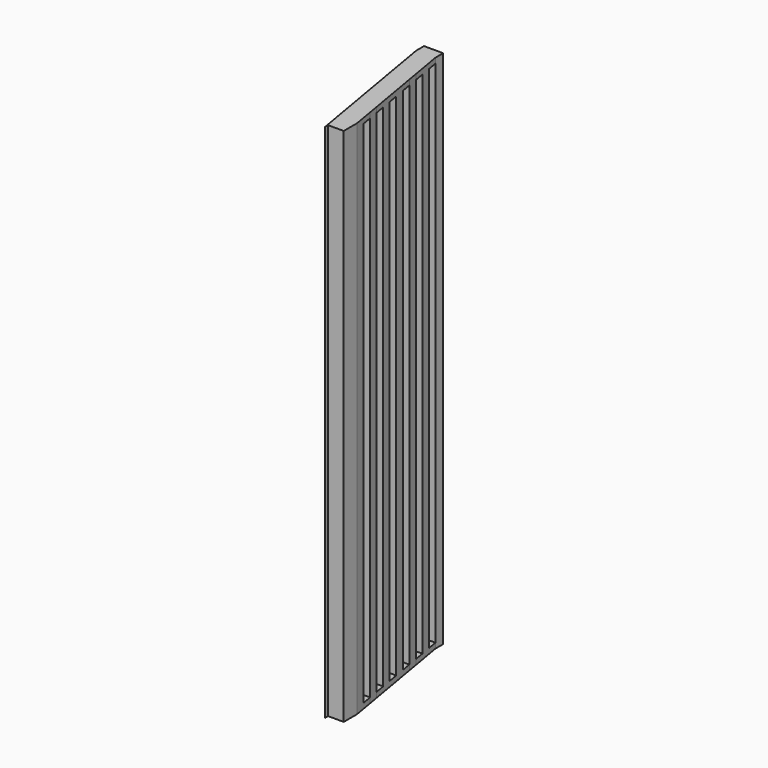
from build123d import *

# Parameters (mm, degrees)
F1_DEPTH = 100
F2_DEPTH = 1
F3_START = 99
F3_DEPTH = 1


with BuildPart() as f1:
    # F0 (on Top) → F1 (new body)
    with BuildSketch(Plane.XY):
        Polygon((-10.3999599814, 2), (-12.5, 2), (-12.5, -1.2), (-9.5, -1.2), (-9.5, 1.1444095289), (-9.5, 2), align=None)
        Polygon((-12.5, -1.2), (-12.5, 2), (-12.8442417498, 4), (-13.5327252493, 4), (-12.5, -2), align=None)
        Polygon((-12.8442417498, 4), (-12.5, 2), (-10.3999599814, 2), (-9.5, 2), (-9.8442417498, 4), align=None)
        Polygon((-13.5327252493, 4), (-12.8442417498, 4), (-13.1884834996, 6), (-13.8769669991, 6), align=None)
        Polygon((-13.5327252493, 8), (-13.1884834996, 6), (-10.1884834996, 6), (-10.5327252493, 8), align=None)
        Polygon((-13.8769669991, 6), (-13.1884834996, 6), (-13.5327252493, 8), (-14.2212087489, 8), align=None)
        Polygon((-14.2212087489, 8), (-13.5327252493, 8), (-13.8769669991, 10), (-14.5654504987, 10), align=None)
        Polygon((-14.2212087489, 12), (-13.8769669991, 10), (-10.8769669991, 10), (-11.2212087489, 12), align=None)
        Polygon((-14.9096922485, 16), (-14.5654504987, 14), (-11.5654504987, 14), (-11.9096922485, 16), align=None)
        Polygon((-15.598175748, 20), (-15.2539339983, 18), (-12.2539339983, 18), (-12.598175748, 20), align=None)
        Polygon((-14.5654504987, 10), (-13.8769669991, 10), (-14.2212087489, 12), (-14.9096922485, 12), align=None)
        Polygon((-14.9096922485, 12), (-14.2212087489, 12), (-14.5654504987, 14), (-15.2539339983, 14), align=None)
        Polygon((-15.2539339983, 14), (-14.5654504987, 14), (-14.9096922485, 16), (-15.598175748, 16), align=None)
        Polygon((-15.598175748, 16), (-14.9096922485, 16), (-15.2539339983, 18), (-15.9424174978, 18), align=None)
        Polygon((-15.9424174978, 18), (-15.2539339983, 18), (-15.598175748, 20), (-16.2866592476, 20), align=None)
        Polygon((-16.2866592476, 20), (-15.598175748, 20), (-15.9424174978, 22), (-16.6309009974, 22), align=None)
        Polygon((-16.6309009974, 22), (-15.9424174978, 22), (-16.2866592476, 24), (-16.9751427472, 24), align=None)
        Polygon((-16.9751427472, 24), (-16.2866592476, 24), (-16.6309009974, 26), (-17.319384497, 26), align=None)
        Polygon((-17.319384497, 26), (-16.6309009974, 26), (-13.6309009974, 26), (-13.6309009974, 27.8660617122), (-17.319384497, 27.8660617122), align=None)
        Polygon((-16.2866592476, 24), (-15.9424174978, 22), (-12.9424174978, 22), (-13.2866592476, 24), align=None)
    extrude(amount=F1_DEPTH)

    # F0 (on Top) → F2 (join)
    with BuildSketch(Plane.XY):
        Polygon((-12.8442417498, 4), (-12.5, 2), (-10.3999599814, 2), (-9.5, 2), (-9.8442417498, 4), align=None)
        Polygon((-12.5, -1.2), (-12.5, 2), (-12.8442417498, 4), (-13.5327252493, 4), (-12.5, -2), align=None)
        Polygon((-13.1884834996, 6), (-12.8442417498, 4), (-9.8442417498, 4), (-10.1884834996, 6), align=None)
        Polygon((-13.5327252493, 4), (-12.8442417498, 4), (-13.1884834996, 6), (-13.8769669991, 6), align=None)
        Polygon((-13.5327252493, 8), (-13.1884834996, 6), (-10.1884834996, 6), (-10.5327252493, 8), align=None)
        Polygon((-13.8769669991, 6), (-13.1884834996, 6), (-13.5327252493, 8), (-14.2212087489, 8), align=None)
        Polygon((-13.8769669991, 10), (-13.5327252493, 8), (-10.5327252493, 8), (-10.8769669991, 10), align=None)
        Polygon((-14.2212087489, 8), (-13.5327252493, 8), (-13.8769669991, 10), (-14.5654504987, 10), align=None)
        Polygon((-14.2212087489, 12), (-13.8769669991, 10), (-10.8769669991, 10), (-11.2212087489, 12), align=None)
        Polygon((-14.5654504987, 10), (-13.8769669991, 10), (-14.2212087489, 12), (-14.9096922485, 12), align=None)
        Polygon((-14.5654504987, 14), (-14.2212087489, 12), (-11.2212087489, 12), (-11.5654504987, 14), align=None)
        Polygon((-14.9096922485, 12), (-14.2212087489, 12), (-14.5654504987, 14), (-15.2539339983, 14), align=None)
        Polygon((-14.9096922485, 16), (-14.5654504987, 14), (-11.5654504987, 14), (-11.9096922485, 16), align=None)
        Polygon((-15.2539339983, 14), (-14.5654504987, 14), (-14.9096922485, 16), (-15.598175748, 16), align=None)
        Polygon((-15.2539339983, 18), (-14.9096922485, 16), (-11.9096922485, 16), (-12.2539339983, 18), align=None)
        Polygon((-15.598175748, 16), (-14.9096922485, 16), (-15.2539339983, 18), (-15.9424174978, 18), align=None)
        Polygon((-15.598175748, 20), (-15.2539339983, 18), (-12.2539339983, 18), (-12.598175748, 20), align=None)
        Polygon((-15.9424174978, 18), (-15.2539339983, 18), (-15.598175748, 20), (-16.2866592476, 20), align=None)
        Polygon((-15.9424174978, 22), (-15.598175748, 20), (-12.598175748, 20), (-12.9424174978, 22), align=None)
        Polygon((-16.2866592476, 20), (-15.598175748, 20), (-15.9424174978, 22), (-16.6309009974, 22), align=None)
        Polygon((-16.2866592476, 24), (-15.9424174978, 22), (-12.9424174978, 22), (-13.2866592476, 24), align=None)
        Polygon((-16.6309009974, 22), (-15.9424174978, 22), (-16.2866592476, 24), (-16.9751427472, 24), align=None)
        Polygon((-16.6309009974, 26), (-16.2866592476, 24), (-13.2866592476, 24), (-13.6309009974, 26), align=None)
        Polygon((-16.9751427472, 24), (-16.2866592476, 24), (-16.6309009974, 26), (-17.319384497, 26), align=None)
        Polygon((-17.319384497, 26), (-16.6309009974, 26), (-13.6309009974, 26), (-13.6309009974, 27.8660617122), (-17.319384497, 27.8660617122), align=None)
    extrude(amount=F2_DEPTH)

    # F0 (on Top) → F3 (join)
    with BuildSketch(Plane.XY.offset(F3_START)):
        Polygon((-12.8442417498, 4), (-12.5, 2), (-10.3999599814, 2), (-9.5, 2), (-9.8442417498, 4), align=None)
        Polygon((-10.3999599814, 2), (-12.5, 2), (-12.5, -1.2), (-9.5, -1.2), (-9.5, 1.1444095289), (-9.5, 2), align=None)
        Polygon((-12.5, -1.2), (-12.5, 2), (-12.8442417498, 4), (-13.5327252493, 4), (-12.5, -2), align=None)
        Polygon((-13.1884834996, 6), (-12.8442417498, 4), (-9.8442417498, 4), (-10.1884834996, 6), align=None)
        Polygon((-13.5327252493, 4), (-12.8442417498, 4), (-13.1884834996, 6), (-13.8769669991, 6), align=None)
        Polygon((-13.5327252493, 8), (-13.1884834996, 6), (-10.1884834996, 6), (-10.5327252493, 8), align=None)
        Polygon((-13.8769669991, 6), (-13.1884834996, 6), (-13.5327252493, 8), (-14.2212087489, 8), align=None)
        Polygon((-13.8769669991, 10), (-13.5327252493, 8), (-10.5327252493, 8), (-10.8769669991, 10), align=None)
        Polygon((-14.2212087489, 8), (-13.5327252493, 8), (-13.8769669991, 10), (-14.5654504987, 10), align=None)
        Polygon((-14.2212087489, 12), (-13.8769669991, 10), (-10.8769669991, 10), (-11.2212087489, 12), align=None)
        Polygon((-14.5654504987, 10), (-13.8769669991, 10), (-14.2212087489, 12), (-14.9096922485, 12), align=None)
        Polygon((-14.5654504987, 14), (-14.2212087489, 12), (-11.2212087489, 12), (-11.5654504987, 14), align=None)
        Polygon((-14.9096922485, 12), (-14.2212087489, 12), (-14.5654504987, 14), (-15.2539339983, 14), align=None)
        Polygon((-14.9096922485, 16), (-14.5654504987, 14), (-11.5654504987, 14), (-11.9096922485, 16), align=None)
        Polygon((-15.2539339983, 14), (-14.5654504987, 14), (-14.9096922485, 16), (-15.598175748, 16), align=None)
        Polygon((-15.2539339983, 18), (-14.9096922485, 16), (-11.9096922485, 16), (-12.2539339983, 18), align=None)
        Polygon((-15.598175748, 16), (-14.9096922485, 16), (-15.2539339983, 18), (-15.9424174978, 18), align=None)
        Polygon((-15.598175748, 20), (-15.2539339983, 18), (-12.2539339983, 18), (-12.598175748, 20), align=None)
        Polygon((-15.9424174978, 18), (-15.2539339983, 18), (-15.598175748, 20), (-16.2866592476, 20), align=None)
        Polygon((-15.9424174978, 22), (-15.598175748, 20), (-12.598175748, 20), (-12.9424174978, 22), align=None)
        Polygon((-16.2866592476, 20), (-15.598175748, 20), (-15.9424174978, 22), (-16.6309009974, 22), align=None)
        Polygon((-16.2866592476, 24), (-15.9424174978, 22), (-12.9424174978, 22), (-13.2866592476, 24), align=None)
        Polygon((-16.6309009974, 22), (-15.9424174978, 22), (-16.2866592476, 24), (-16.9751427472, 24), align=None)
        Polygon((-16.6309009974, 26), (-16.2866592476, 24), (-13.2866592476, 24), (-13.6309009974, 26), align=None)
        Polygon((-16.9751427472, 24), (-16.2866592476, 24), (-16.6309009974, 26), (-17.319384497, 26), align=None)
        Polygon((-17.319384497, 26), (-16.6309009974, 26), (-13.6309009974, 26), (-13.6309009974, 27.8660617122), (-17.319384497, 27.8660617122), align=None)
    extrude(amount=F3_DEPTH)


solid = f1.part
